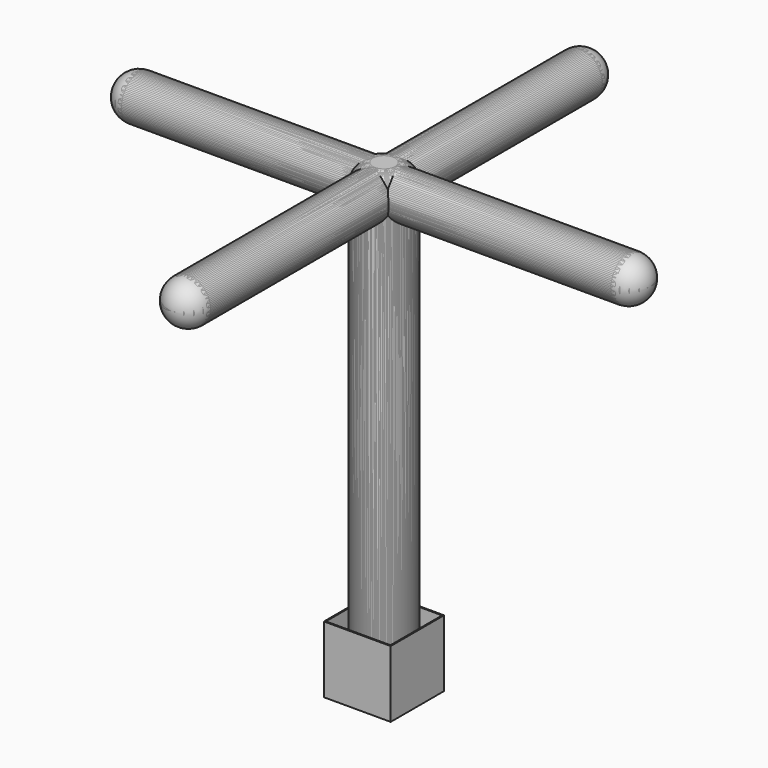
from build123d import *

# Parameters (mm, degrees)
F0_W      = 152.4
F0_H      = 152.4
F1_DEPTH  = 152.4
F2_T      = -2.54
F3_R      = 63.5
F6_R      = 63.5
F9_R      = 50.8
F10_DEPTH = 609.6
F11_R     = 50.8
F12_COUNT = 4


# Not quite as in the source:
# - a fillet or chamfer that OpenCascade refuses, or shapes differently, is made with other operations: its cross-section is extruded or revolved along the edge and cut away or added


with BuildPart() as f1:
    # F0 (on Top) → F1 (new body)
    with BuildSketch(Plane.XY):
        Rectangle(F0_W, F0_H)
    extrude(amount=F1_DEPTH)

    # F2
    f2_openings = [f1.faces().sort_by_distance(p)[0] for p in [
        (0, 0, 152.4),
    ]]
    offset(amount=F2_T, openings=f2_openings)

    # F3 (on face) → F7 section 0
    with BuildSketch(Plane.XY.offset(2.54)):
        Circle(F3_R)
    # F6 (on offset) → F7 section 1
    with BuildSketch(Plane.XY.offset(1069.34)):
        Circle(F6_R)
    loft()

    # F8: fillet of radius 38.1 on 3 edges, made by hand


with BuildPart() as f8_tool2:
    # F8_s3 → F8_t4 (revolve)
    with BuildSketch(Plane.XZ):
        with BuildLine():
            ThreePointArc((101.6, 2.54), (74.6592316368, 13.6992316368), (63.5, 40.64))
            Line((63.5, 40.64), (63.5, 2.54))
            Line((63.5, 2.54), (101.6, 2.54))
        make_face()
    revolve(axis=Axis((0, 0, 2.54), (0, 0, 1)))

    split(bisect_by=Plane.YZ.offset(73.66), keep=Keep.BOTTOM)

    split(bisect_by=Plane.XZ.offset(73.66), keep=Keep.BOTTOM)

    split(bisect_by=Plane.YZ.offset(-73.66), keep=Keep.TOP)

    split(bisect_by=Plane.XZ.offset(-73.66), keep=Keep.TOP)


with BuildPart() as f1_1:
    add(f1.part)

    # F8_t1: union F8_tool2
    add(f8_tool2.part)

    # F8_s9 → F8_t10 (revolve, cut)
    with BuildSketch(Plane.XZ):
        with BuildLine():
            ThreePointArc((63.5, 1031.24), (52.3407683632, 1058.1807683632), (25.4, 1069.34))
            Line((25.4, 1069.34), (63.5, 1069.34))
            Line((63.5, 1069.34), (63.5, 1031.24))
        make_face()
    revolve(axis=Axis((0, 0, 1069.34), (0, 0, 1)), mode=Mode.SUBTRACT)

    # F9 (on Right) → F10 (join, symmetric)
    with BuildSketch(Plane.YZ):
        with Locations((0, 1018.54)):
            Circle(F9_R)
    extrude(amount=F10_DEPTH, both=True)

    # F11
    f11_edges = [f1_1.edges().sort_by_distance(p)[0] for p in [
        (-609.6, -50.8, 1018.54),
        (609.6, -50.8, 1018.54),
    ]]
    fillet(f11_edges, radius=F11_R)


with BuildPart() as f12_1:
    # F12: instance of F1
    add(f1_1.part.rotate(Axis((0, 0, 533.4), (0, 0, 1)), 1 * 360 / F12_COUNT))


with BuildPart() as f12_2:
    # F12: instance of F1
    add(f1_1.part.rotate(Axis((0, 0, 533.4), (0, 0, 1)), 2 * 360 / F12_COUNT))


with BuildPart() as f12_3:
    # F12: instance of F1
    add(f1_1.part.rotate(Axis((0, 0, 533.4), (0, 0, 1)), 3 * 360 / F12_COUNT))


solid = Compound([f1_1.part, f12_1.part, f12_2.part, f12_3.part])
